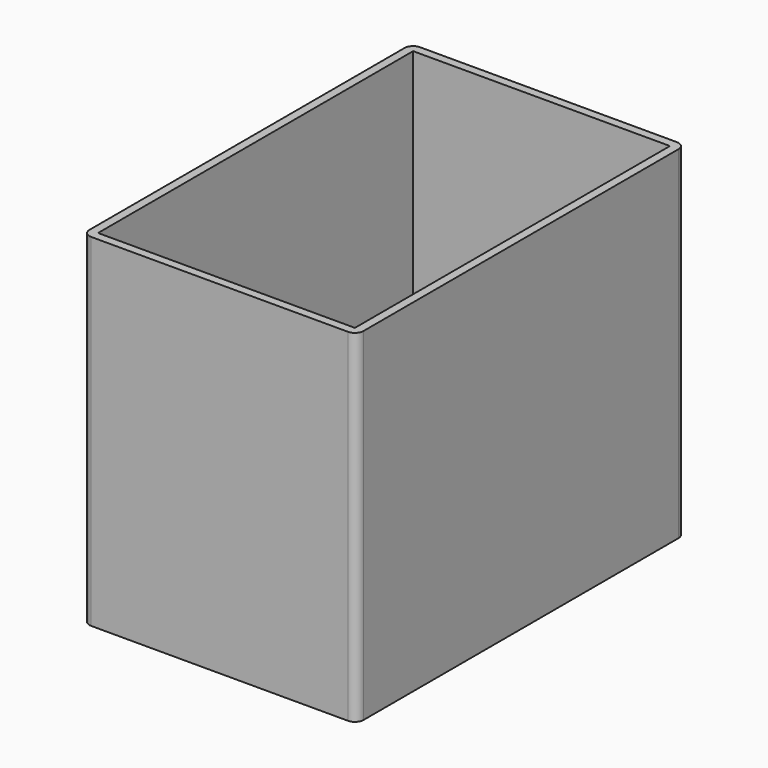
from build123d import *

# Parameters (mm, degrees)
F1_DEPTH = 127
F2_T     = 3.175


# Not quite as in the source:
# - a shell that OpenCascade refuses in one call is made with other operations: the cavity is built on its own and cut out


with BuildPart() as f1:
    # F0 (on Top) → F1 (new body)
    with BuildSketch(Plane.XY):
        with BuildLine():
            ThreePointArc((50.8, 73.025), (49.8700640303, 75.2700640303), (47.625, 76.2))
            Line((47.625, 76.2), (-47.625, 76.2))
            ThreePointArc((-47.625, 76.2), (-49.8700640303, 75.2700640303), (-50.8, 73.025))
            Line((-50.8, 73.025), (-50.8, -73.025))
            ThreePointArc((-50.8, -73.025), (-49.8700640303, -75.2700640303), (-47.625, -76.2))
            Line((-47.625, -76.2), (47.625, -76.2))
            ThreePointArc((47.625, -76.2), (49.8700640303, -75.2700640303), (50.8, -73.025))
            Line((50.8, -73.025), (50.8, 73.025))
        make_face()
    extrude(amount=F1_DEPTH)

    # F2: shell of thickness 3.175, made by hand


with BuildPart() as f2_core1:
    # F2_t2: copy of F1
    add(f1.part)

    # the walls: a layer under each face that stays
    f2_faces = [f2_core1.faces().sort_by_distance(p)[0] for p in [
        (0, 76.2, 63.5),
        (-50.8, 0, 63.5),
        (0, -76.2, 63.5),
        (50.8, 0, 63.5),
        (0, 0, 0),
    ]]
    thicken(f2_faces, amount=-F2_T, mode=Mode.SUBTRACT)


with BuildPart() as f1_1:
    add(f1.part)

    # what is left inside the walls is the cavity
    f2_cavity = [f2_core1.part.solids().sort_by_distance(p)[0] for p in [
        (47.59325, 0, 85.725),
    ]]
    add(f2_cavity, mode=Mode.SUBTRACT)


solid = f1_1.part
